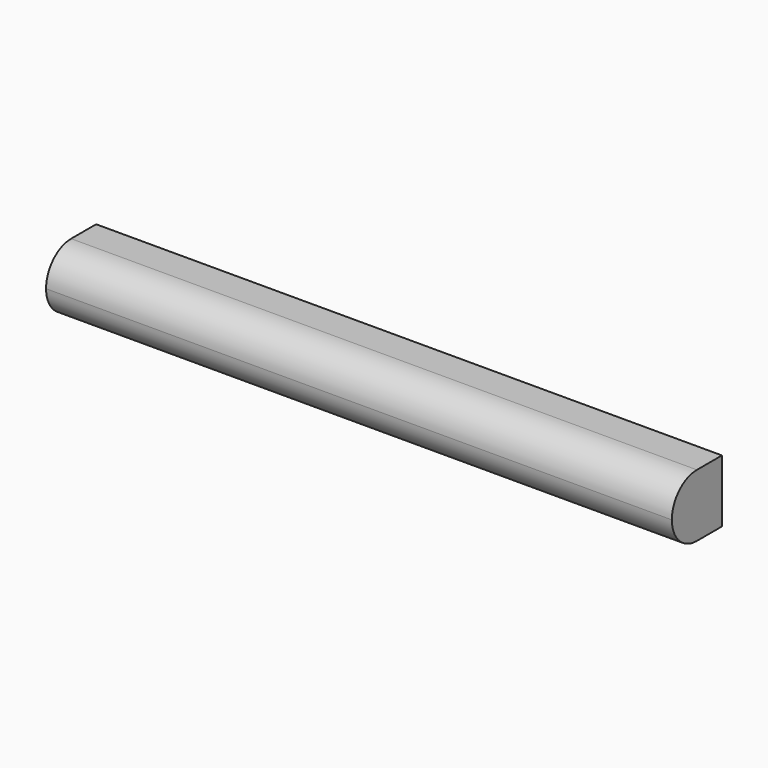
from build123d import *

# Parameters (mm, degrees)
F0_W     = 100
F0_H     = 10
F1_DEPTH = 10
F2_R     = 4.99999


# Not quite as in the source:
# - a fillet or chamfer is up to 0.001 mm smaller than in the source, because OpenCascade refuses the exact size


with BuildPart() as f1:
    # F0 (on Front) → F1 (new body)
    with BuildSketch(Plane.XZ):
        Rectangle(F0_W, F0_H)
    extrude(amount=F1_DEPTH)

    # F2 (radius 5 in the source; OpenCascade refuses exactly that, so slightly less here)
    f2_edges = [f1.edges().sort_by_distance(p)[0] for p in [
        (0, -10, -5),
        (0, -10, 5),
    ]]
    fillet(f2_edges, radius=F2_R)


solid = f1.part
